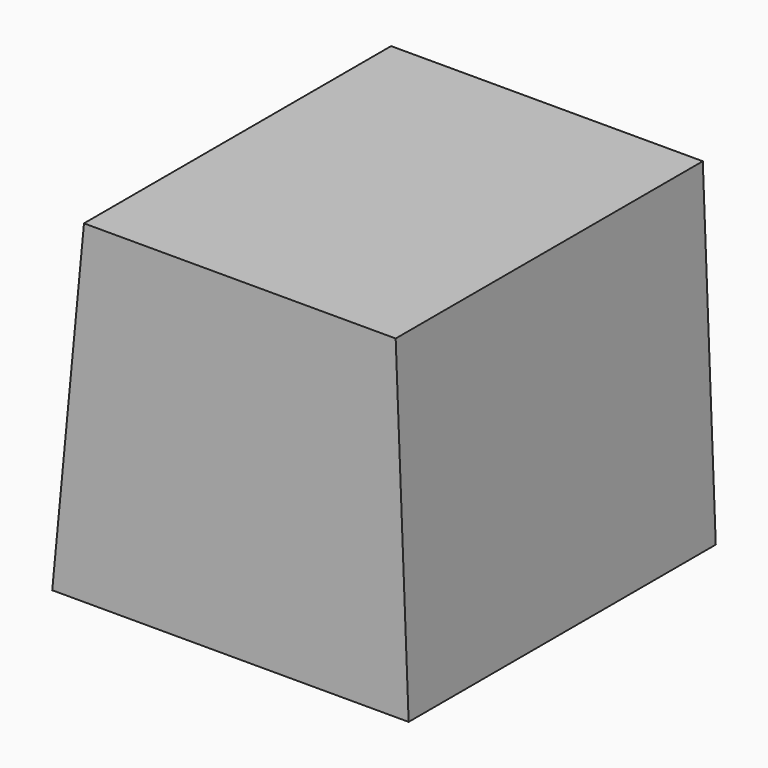
from build123d import *

# Parameters (mm, degrees)
F1_DEPTH = 25
F3_DEPTH = 25


# Not quite as in the source:
# - the program builds the solid bodies; features that only make, move or delete a surface that nothing else refers to are left out


with BuildPart() as f1:
    # F0 (on Front) → F1 (new body)
    with BuildSketch(Plane.XZ):
        Polygon((20.8621732891, 24.997016415), (-19.7344869375, 24.997016415), (-23.8693337888, -18.4188559651), (22.5537028164, -18.4188559651), align=None)
    extrude(amount=F1_DEPTH)

    # F3 (add): a face of the model
    f3_faces = [f1.faces().sort_by_distance(p)[0] for p in [
        (-0.0606187837, -25, 2.8045975494),
    ]]
    extrude(f3_faces, amount=F3_DEPTH)


solid = f1.part
